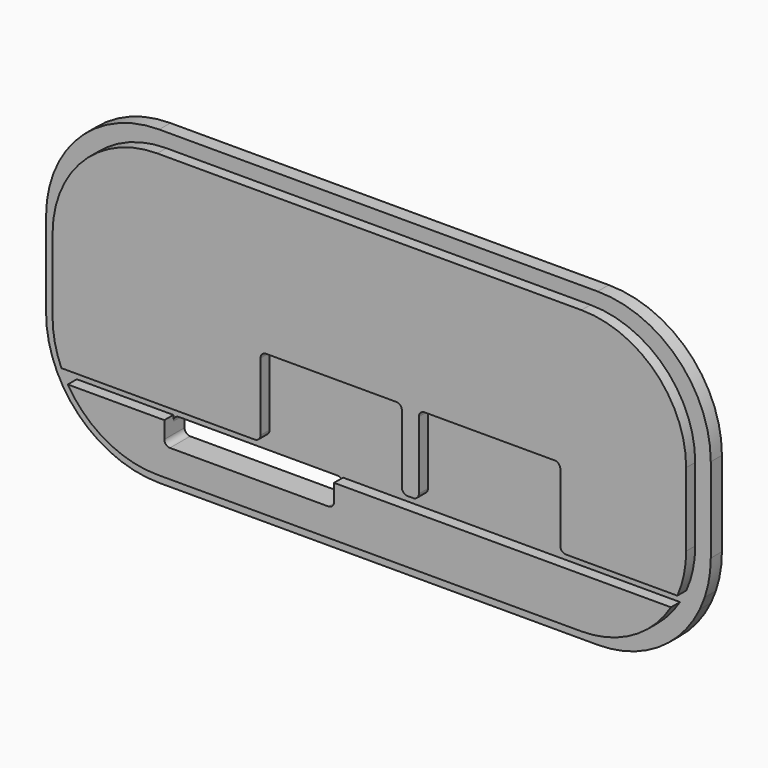
from build123d import *

# Parameters (mm, degrees)
F1_DEPTH = 1.25222
F3_DEPTH = 1.016
F4_W     = 12.7
F4_H     = 7.112
F5_DEPTH = 1.016
F6_W     = 15.24
F6_H     = 2.032
F7_DEPTH = 25.4
F8_R     = 0.508


with BuildPart() as f1:
    # F0 (on Front) → F1 (new body)
    with BuildSketch(Plane.XZ):
        with BuildLine():
            Line((27.6567419321, -7.07644), (29.3056013183, -7.07644))
            ThreePointArc((29.3056013183, -7.07644), (29.7092433479, -5.4653384255), (29.845, -3.81))
            Line((29.845, -3.81), (29.845, 3.81))
            ThreePointArc((29.845, 3.81), (26.8692048969, 10.9942048969), (19.685, 13.97))
            Line((19.685, 13.97), (-19.685, 13.97))
            ThreePointArc((-19.685, 13.97), (-26.8692048969, 10.9942048969), (-29.845, 3.81))
            Line((-29.845, 3.81), (-29.845, -3.81))
            ThreePointArc((-29.845, -3.81), (-29.7092433479, -5.4653384255), (-29.3056013183, -7.07644))
            Line((-29.3056013183, -7.07644), (-27.6567419321, -7.07644))
            ThreePointArc((-27.6567419321, -7.07644), (-28.2480586179, -5.230243154), (-28.448, -3.302))
            Line((-28.448, -3.302), (-28.448, 3.302))
            ThreePointArc((-28.448, 3.302), (-25.6953895296, 9.9473895296), (-19.05, 12.7))
            Line((-19.05, 12.7), (19.05, 12.7))
            ThreePointArc((19.05, 12.7), (25.6953895296, 9.9473895296), (28.448, 3.302))
            Line((28.448, 3.302), (28.448, -3.302))
            ThreePointArc((28.448, -3.302), (28.2480586179, -5.230243154), (27.6567419321, -7.07644))
        make_face()
        with BuildLine():
            Line((-19.685, -13.97), (19.685, -13.97))
            ThreePointArc((19.685, -13.97), (25.1077661576, -12.4018104728), (28.8565313119, -8.18134))
            Line((28.8565313119, -8.18134), (27.0820884684, -8.18134))
            ThreePointArc((27.0820884684, -8.18134), (23.6579478448, -11.4928009779), (19.05, -12.7))
            Line((19.05, -12.7), (-19.05, -12.7))
            ThreePointArc((-19.05, -12.7), (-23.6579478448, -11.4928009779), (-27.0820884684, -8.18134))
            Line((-27.0820884684, -8.18134), (-28.8565313119, -8.18134))
            ThreePointArc((-28.8565313119, -8.18134), (-25.1077661576, -12.4018104728), (-19.685, -13.97))
        make_face()
        with BuildLine():
            Line((-29.3056013183, -7.07644), (-28.8565313119, -8.18134))
            Line((-28.8565313119, -8.18134), (-27.0820884684, -8.18134))
            ThreePointArc((-27.0820884684, -8.18134), (-27.3877377194, -7.6384194588), (-27.6567419321, -7.07644))
            Line((-27.6567419321, -7.07644), (-29.3056013183, -7.07644))
        make_face()
        with BuildLine():
            Line((27.0820884684, -8.18134), (28.8565313119, -8.18134))
            Line((28.8565313119, -8.18134), (29.3056013183, -7.07644))
            Line((29.3056013183, -7.07644), (27.6567419321, -7.07644))
            ThreePointArc((27.6567419321, -7.07644), (27.3877377194, -7.6384194588), (27.0820884684, -8.18134))
        make_face()
        with BuildLine():
            Line((-27.6567419321, -7.07644), (27.6567419321, -7.07644))
            ThreePointArc((27.6567419321, -7.07644), (28.2480586179, -5.230243154), (28.448, -3.302))
            Line((28.448, -3.302), (28.448, 3.302))
            ThreePointArc((28.448, 3.302), (25.6953895296, 9.9473895296), (19.05, 12.7))
            Line((19.05, 12.7), (-19.05, 12.7))
            ThreePointArc((-19.05, 12.7), (-25.6953895296, 9.9473895296), (-28.448, 3.302))
            Line((-28.448, 3.302), (-28.448, -3.302))
            ThreePointArc((-28.448, -3.302), (-28.2480586179, -5.230243154), (-27.6567419321, -7.07644))
        make_face()
        with BuildLine():
            Line((-27.0820884684, -8.18134), (27.0820884684, -8.18134))
            ThreePointArc((27.0820884684, -8.18134), (27.3877377194, -7.6384194588), (27.6567419321, -7.07644))
            Line((27.6567419321, -7.07644), (-27.6567419321, -7.07644))
            ThreePointArc((-27.6567419321, -7.07644), (-27.3877377194, -7.6384194588), (-27.0820884684, -8.18134))
        make_face()
        with BuildLine():
            ThreePointArc((19.05, -12.7), (23.6579478448, -11.4928009779), (27.0820884684, -8.18134))
            Line((27.0820884684, -8.18134), (-27.0820884684, -8.18134))
            ThreePointArc((-27.0820884684, -8.18134), (-23.6579478448, -11.4928009779), (-19.05, -12.7))
            Line((-19.05, -12.7), (19.05, -12.7))
        make_face()
    extrude(amount=F1_DEPTH)

    # F2 (on face) → F3 (join)
    with BuildSketch(Plane.XZ.offset(1.25222)):
        with BuildLine():
            Line((-19.05, -12.7), (19.05, -12.7))
            ThreePointArc((19.05, -12.7), (23.6579478448, -11.4928009779), (27.0820884684, -8.18134))
            Line((27.0820884684, -8.18134), (-27.0820884684, -8.18134))
            ThreePointArc((-27.0820884684, -8.18134), (-23.6579478448, -11.4928009779), (-19.05, -12.7))
        make_face()
        with BuildLine():
            Line((-27.6567419321, -7.07644), (27.6567419321, -7.07644))
            ThreePointArc((27.6567419321, -7.07644), (28.2480586179, -5.230243154), (28.448, -3.302))
            Line((28.448, -3.302), (28.448, 3.302))
            ThreePointArc((28.448, 3.302), (25.6953895296, 9.9473895296), (19.05, 12.7))
            Line((19.05, 12.7), (-19.05, 12.7))
            ThreePointArc((-19.05, 12.7), (-25.6953895296, 9.9473895296), (-28.448, 3.302))
            Line((-28.448, 3.302), (-28.448, -3.302))
            ThreePointArc((-28.448, -3.302), (-28.2480586179, -5.230243154), (-27.6567419321, -7.07644))
        make_face()
    extrude(amount=F3_DEPTH)

    # F4 (on face) → F5 (cut)
    with BuildSketch(Plane.XZ.offset(2.26822)):
        with Locations((-3.429, -3.52044)):
            Rectangle(F4_W, F4_H)
        with Locations((10.795, -3.52044)):
            Rectangle(F4_W, F4_H)
    extrude(amount=-F5_DEPTH, mode=Mode.SUBTRACT)

    # F6 (on face) → F7 (cut)
    with BuildSketch(Plane.XZ.offset(2.26822)):
        with Locations((-10.795, -9.19734)):
            Rectangle(F6_W, F6_H)
    extrude(amount=-F7_DEPTH, mode=Mode.SUBTRACT)

    # F8
    f8_edges = [f1.edges().sort_by_distance(p)[0] for p in [
        (17.145, -1.76022, -7.07644),
        (17.145, -1.76022, 0.03556),
        (4.445, -1.76022, -7.07644),
        (4.445, -1.76022, 0.03556),
        (-9.779, -1.76022, 0.03556),
        (2.921, -1.76022, 0.03556),
        (2.921, -1.76022, -7.07644),
        (-9.779, -1.76022, -7.07644),
        (-3.175, -1.13411, -10.21334),
        (-18.415, -0.62611, -8.18134),
        (-18.415, -1.13411, -10.21334),
        (-3.175, -0.62611, -8.18134),
    ]]
    fillet(f8_edges, radius=F8_R)


solid = f1.part
